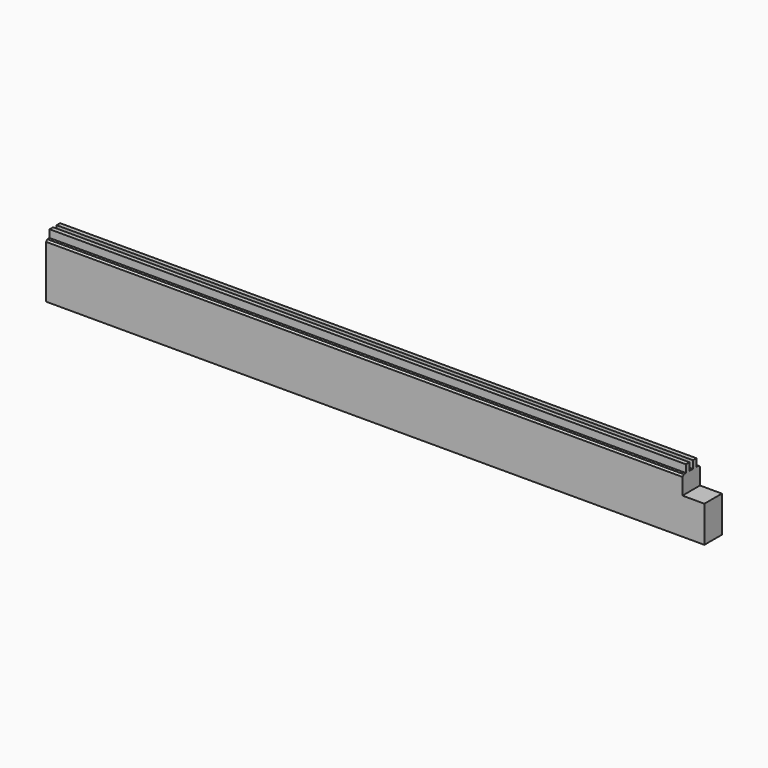
from build123d import *

# Parameters (mm, degrees)
F1_W     = 40
F1_H     = 33
F3_DEPTH = 600
F2_W     = 80
F2_H     = 100
F4_DEPTH = 25
F5_W     = 1200
F5_H     = 50
F6_DEPTH = 1235


# Not quite as in the source:
# - an extrude ends at something that could not be found from the text; its depth is read off the source's solid


with BuildPart() as f3:
    # F1 (on Right) → F3 (new body, symmetric)
    with BuildSketch(Plane.YZ):
        Polygon((20, 33), (20, 63), (17, 66), (12, 66), (12, 80), (4, 80), (4, 66), (-4, 66), (-4, 80), (-12, 80), (-12, 66), (-17, 66), (-20, 63), (-20, 33), align=None)
        with Locations((0, 16.5)):
            Rectangle(F1_W, F1_H)
        with Locations((0, -16.5)):
            Rectangle(F1_W, F1_H)
    extrude(amount=F3_DEPTH, both=True)

    # F2 (on Front) → F4 (cut, symmetric)
    with BuildSketch(Plane.XZ):
        with Locations((600, 83)):
            Rectangle(F2_W, F2_H)
        with Locations((600, -83)):
            Rectangle(F2_W, F2_H)
    extrude(amount=F4_DEPTH, both=True, mode=Mode.SUBTRACT)

    # F5 (on face) → F6 (cut, through all)
    with BuildSketch(Plane.XZ.offset(20)):
        with Locations((0, -58)):
            Rectangle(F5_W, F5_H)
    extrude(amount=-F6_DEPTH, mode=Mode.SUBTRACT)


solid = f3.part
